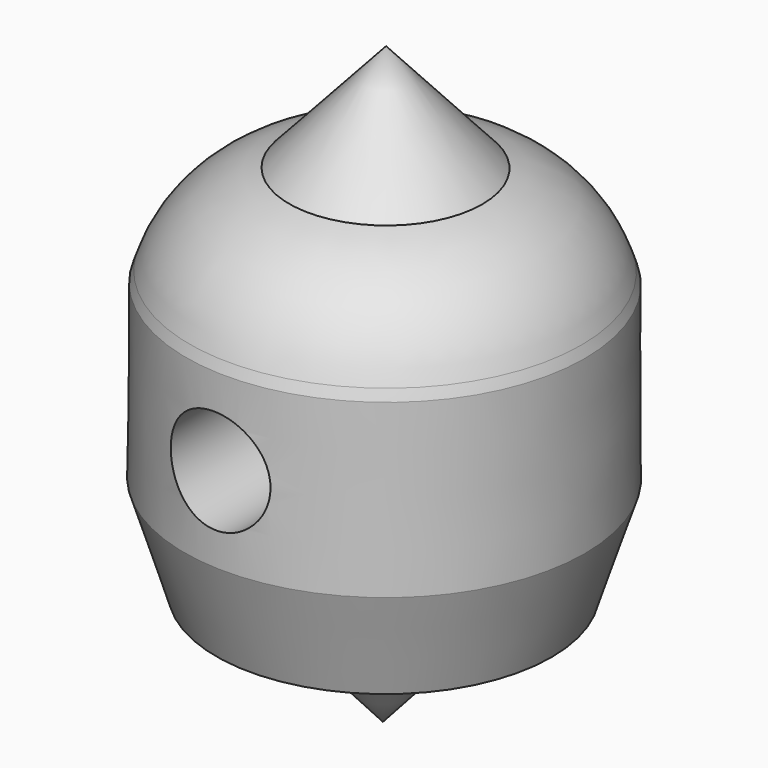
from build123d import *

# Parameters (mm, degrees)
F2_R          = 7.4871337732
F3_DEPTH      = 38.4
F3_DEPTH_BACK = 28.9757450369


# Not quite as in the source:
# - a fillet or chamfer that OpenCascade refuses, or shapes differently, is made with other operations: its cross-section is extruded or revolved along the edge and cut away or added


with BuildPart() as f1:
    # F0 (on Front) → F1 (revolve)
    with BuildSketch(Plane.XZ):
        Polygon((-10.0024826825, 27.1807126701), (-23.9010660062, 42.7652467351), (-24.3538618088, -43.2729683816), (-10.0024826825, -27.1807126701), (0, -27.1280723152), (4.7837961465, -12.3932333663), (4.7837961465, 0), (4.7837961465, 12.3932333663), (0, 27.1280723152), align=None)
    revolve(axis=Axis((-24.1274639075, 0, -0.2538608233), (-0.005262656, 0, -0.9999861521)))

    # F2 (on Front) → F3 (cut, two sides)
    with BuildSketch(Plane.XZ) as f3_sk:
        with Locations((-25.4709236324, 0)):
            Circle(F2_R)
    extrude(amount=-F3_DEPTH, mode=Mode.SUBTRACT)
    extrude(f3_sk.sketch, amount=F3_DEPTH_BACK, mode=Mode.SUBTRACT)

    # F4: fillet of radius 20 on 1 edges, made by hand

    # F4_s1 → F4_t2 (revolve, cut)
    with BuildSketch(Plane.XZ):
        with BuildLine():
            ThreePointArc((4.2865600872, 13.9247980545), (-1.133885263, 22.4112009628), (-10.0024826825, 27.1807126701))
            Line((-10.0024826825, 27.1807126701), (-9.9078117783, 27.5693480003))
            ThreePointArc((-9.9078117783, 27.5693480003), (-4.9991362788, 27.5543869535), (0.0021050624, 27.5280667761))
            Line((0.0021050624, 27.5280667761), (0.3804517595, 27.2515893532))
            Line((0.3804517595, 27.2515893532), (4.6670118467, 14.0483150925))
            Line((4.6670118467, 14.0483150925), (4.2865600872, 13.9247980545))
        make_face()
    revolve(axis=Axis((-23.9826959839, 0, 27.2542867429), (-0.005262656, 0, -0.9999861521)), mode=Mode.SUBTRACT)


solid = f1.part
